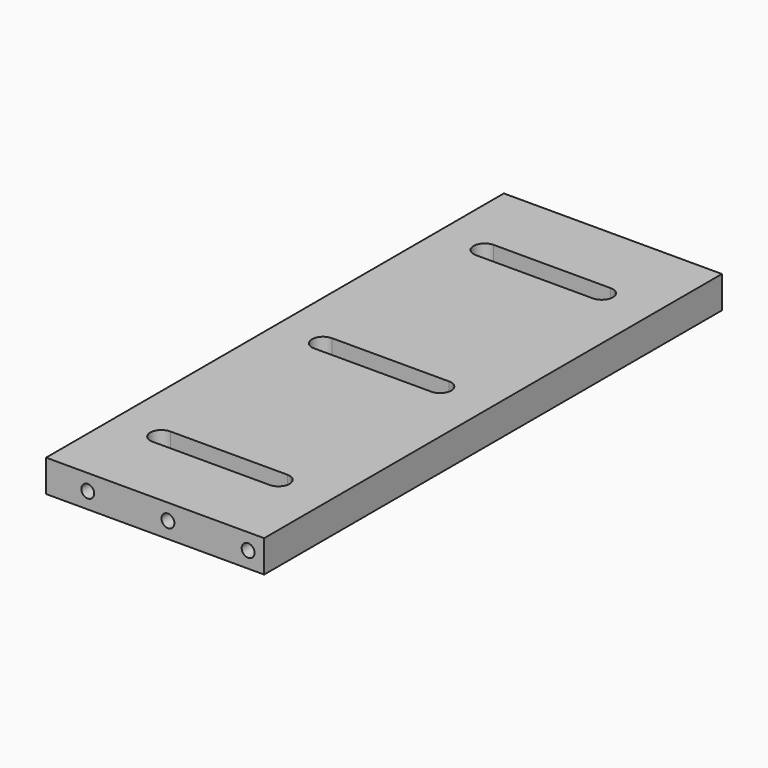
from build123d import *

# Parameters (mm, degrees)
F0_W     = 86.36
F0_H     = 12.7
F1_DEPTH = 226.6
F3_D     = 8.8
F6_D     = 5.1054
F6_DEPTH = 15.875
F6_TIP   = 1.5338169022
F8_D     = 5.1054
F8_DEPTH = 15.875
F8_TIP   = 1.5338169022
F9_DEPTH = 25.4


# Not quite as in the source:
# - a feature names something its author has since deleted; it is built from what else it names


with BuildPart() as f1:
    # F0 (on Front) → F1 (new body)
    with BuildSketch(Plane.XZ):
        with Locations((43.18, 6.35)):
            Rectangle(F0_W, F0_H)
    extrude(amount=F1_DEPTH)

    # F3 (through all)
    with Locations(Plane.XY.offset(12.7)):
        with Locations((19.05, -113.29949), (65.405, -113.29949), (65.405, -33.28949), (19.05, -193.30949), (65.405, -193.30949), (19.05, -33.28949)):
            Hole(F3_D / 2)

    # F6
    with Locations(Plane.XZ.offset(226.6)):
        with Locations((16.51, 6.35), (48.26, 6.35), (80.01, 6.35)):
            Hole(F6_D / 2, depth=F6_DEPTH)
            with Locations((0, 0, -(F6_DEPTH + F6_TIP / 2))):  # 118° drill point
                Cone(0, F6_D / 2, F6_TIP, mode=Mode.SUBTRACT)

    # F8
    with Locations(Plane(origin=(0, 0, 0), x_dir=(-1, 0, 0), z_dir=(0, 1, 0))):
        with Locations((-80.01, 6.35), (-48.26, 6.35), (-16.51, 6.35)):
            Hole(F8_D / 2, depth=F8_DEPTH)
            with Locations((0, 0, -(F8_DEPTH + F8_TIP / 2))):  # 118° drill point
                Cone(0, F8_D / 2, F8_TIP, mode=Mode.SUBTRACT)

    # F4 (on face) → F9 (cut)
    with BuildSketch(Plane.XY.offset(12.7)):
        with BuildLine():
            ThreePointArc((23.45, -193.30949), (22.1612698372, -196.4207598372), (19.05, -197.70949))
            Line((19.05, -197.70949), (65.405, -197.70949))
            ThreePointArc((65.405, -197.70949), (61.005, -193.30949), (65.405, -188.90949))
            Line((65.405, -188.90949), (19.05, -188.90949))
            ThreePointArc((19.05, -188.90949), (22.1612698372, -190.1982201628), (23.45, -193.30949))
        make_face()
        with BuildLine():
            ThreePointArc((65.405, -117.69949), (61.005, -113.29949), (65.405, -108.89949))
            Line((65.405, -108.89949), (19.05, -108.89949))
            ThreePointArc((19.05, -108.89949), (22.1612698372, -110.1882201628), (23.45, -113.29949))
            ThreePointArc((23.45, -113.29949), (22.1612698372, -116.4107598372), (19.05, -117.69949))
            Line((19.05, -117.69949), (65.405, -117.69949))
        make_face()
        with BuildLine():
            ThreePointArc((65.405, -37.68949), (61.005, -33.28949), (65.405, -28.88949))
            Line((65.405, -28.88949), (19.05, -28.88949))
            ThreePointArc((19.05, -28.88949), (22.1612698372, -30.1782201628), (23.45, -33.28949))
            ThreePointArc((23.45, -33.28949), (22.1612698372, -36.4007598372), (19.05, -37.68949))
            Line((19.05, -37.68949), (65.405, -37.68949))
        make_face()
    extrude(amount=-F9_DEPTH, mode=Mode.SUBTRACT)


solid = f1.part
